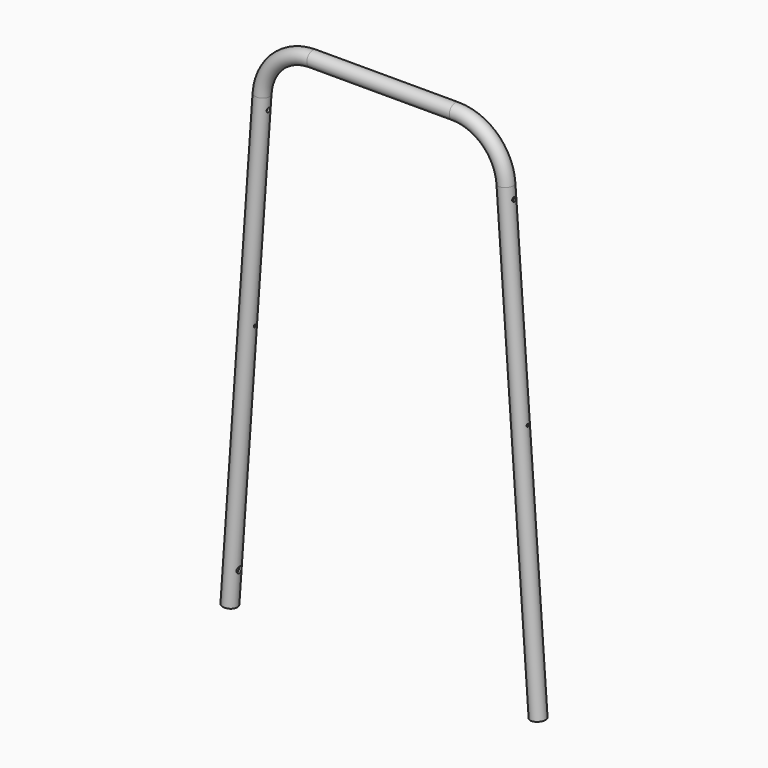
from build123d import *

# Parameters (mm, degrees)
F3_R          = 11.1125
F3_R_2        = 7.9375
F6_R          = 4.7625
F7_DEPTH      = 25.4
F8_R          = 3.175
F8_R_2        = 1.9812
F9_DEPTH      = 25.4
F9_DEPTH_BACK = 25.4


# Not quite as in the source:
# - a feature of the source that left no trace in its solid (it failed there, or was rolled back) is left out
# - a pattern or mirror of a feature is missing from the dataset's text; its kind, count and spacing are read off the source's solid


with BuildPart() as f4:
    # F4: sweep along a path in F1
    with BuildLine(Plane.XZ.offset(406.4)) as f4_path:
        Line((-256.354432993, -633.143806298), (-208.1567310661, 56.1154432993))
        ThreePointArc((-208.1567310661, 56.1154432993), (-184.1106254731, 106.5291520634), (-132.1423504363, 127))
        Line((-132.1423504363, 127), (81.3423504363, 127))
        ThreePointArc((81.3423504363, 127), (133.3106254731, 106.5291520634), (157.3567310661, 56.1154432993))
        Line((157.3567310661, 56.1154432993), (205.554432993, -633.143806298))
    # F3 (on line) → F4 (sweep)
    with BuildSketch(Plane(origin=(-45.3057052979, 0, -647.9017709904), x_dir=(0.9975640503, 0, -0.0697564737), z_dir=(-0.0697564737, 0, -0.9975640503))):
        with Locations((-211.5640871783, 406.4)):
            Circle(F3_R)
        with Locations((-211.5640871783, 406.4)):
            Circle(F3_R_2, mode=Mode.SUBTRACT)
    sweep(path=f4_path.line)

    # F6 (on line) → F7 (cut)
    with BuildSketch(Plane(origin=(-211.0487276951, 0, 14.7579646925), x_dir=(0, -1, 0), z_dir=(-0.9975640503, 0, 0.0697564737))):
        with Locations((406.4, -598.6838810818)):
            Circle(F6_R)
    f7 = extrude(amount=-F7_DEPTH, mode=Mode.SUBTRACT)

    # F7_copies: F7 across plane
    add(f7.mirror(Plane(origin=(-25.399975, 2e-06, 1e-06), x_dir=(0, 0, 1), z_dir=(1, 0, 0))), mode=Mode.SUBTRACT)

    # F8 (on line) → F9 (cut, two sides)
    with BuildSketch(Plane(origin=(-211.0487276951, 0, 14.7579646925), x_dir=(0, -1, 0), z_dir=(-0.9975640503, 0, 0.0697564737))) as f9_sk:
        with Locations((406.4, 23.6784693545)):
            Circle(F8_R)
        with Locations((406.4, -268.4215306455)):
            Circle(F8_R_2)
    f9 = extrude(amount=-F9_DEPTH, mode=Mode.SUBTRACT) + extrude(f9_sk.sketch, amount=F9_DEPTH_BACK, mode=Mode.SUBTRACT)

    # F9_copies: F9 across plane
    add(f9.mirror(Plane(origin=(-25.400012, 0, 1e-06), x_dir=(0, 0, 1), z_dir=(1, 0, 0))), mode=Mode.SUBTRACT)


solid = f4.part
